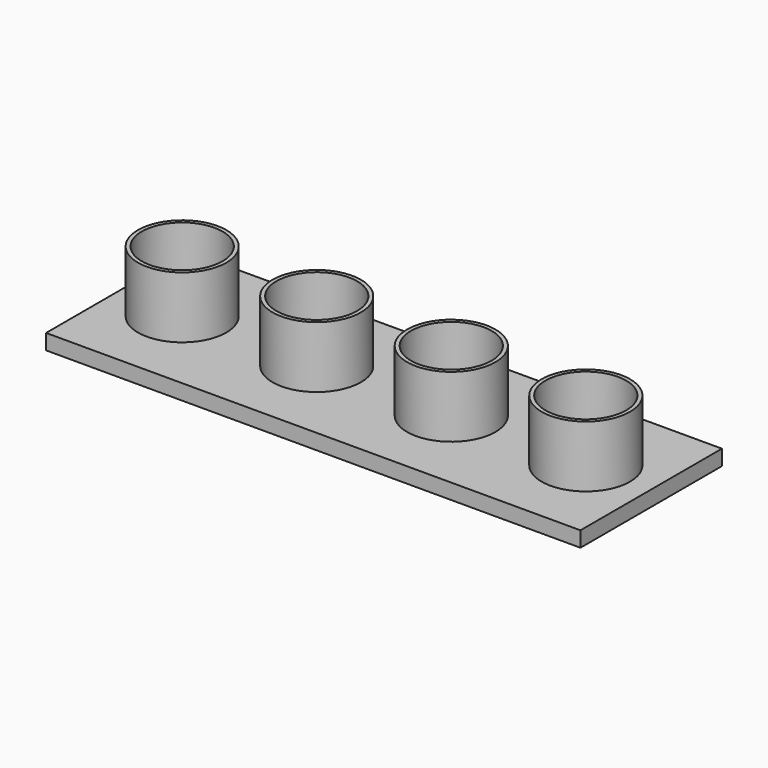
from build123d import *

# Parameters (mm, degrees)
F0_W     = 69.5
F0_H     = 23
F0_R     = 5.75
F0_W_2   = 1
F0_H_2   = 4
F1_DEPTH = 2
F0_R_2   = 5.25
F2_DEPTH = 10


with BuildPart() as f1:
    # F0 (on Top) → F1 (new body)
    with BuildSketch(Plane.XY):
        with Locations((3.4471642077, -3.0003356891)):
            Rectangle(F0_W, F0_H)
        Polygon((-29.8028357923, -13.0003356891), (-29.8028357923, 6.9996643109), (-15.8028357923, 6.9996643109), (-14.8028357923, 6.9996643109), (-13.3028357923, 6.9996643109), (-12.3028357923, 6.9996643109), (1.6971642077, 6.9996643109), (2.6971642077, 6.9996643109), (4.1971642077, 6.9996643109), (5.1971642077, 6.9996643109), (19.1971642077, 6.9996643109), (20.1971642077, 6.9996643109), (21.6971642077, 6.9996643109), (22.6971642077, 6.9996643109), (36.6971642077, 6.9996643109), (36.6971642077, -13.0003356891), (22.6971642077, -13.0003356891), (21.6971642077, -13.0003356891), (20.1971642077, -13.0003356891), (19.1971642077, -13.0003356891), (5.1971642077, -13.0003356891), (5.1971642077, -9.0003356891), (4.1971642077, -9.0003356891), (4.1971642077, -13.0003356891), (2.6971642077, -13.0003356891), (1.6971642077, -13.0003356891), (-12.3028357923, -13.0003356891), (-13.3028357923, -13.0003356891), (-14.8028357923, -13.0003356891), (-15.8028357923, -13.0003356891), align=None, mode=Mode.SUBTRACT)
        Polygon((-15.8028357923, 6.9996643109), (-29.8028357923, 6.9996643109), (-29.8028357923, -13.0003356891), (-15.8028357923, -13.0003356891), (-15.8028357923, -9.0003356891), (-14.8028357923, -9.0003356891), (-14.8028357923, -13.0003356891), (-13.3028357923, -13.0003356891), (-13.3028357923, -9.0003356891), (-12.3028357923, -9.0003356891), (-12.3028357923, -13.0003356891), (1.6971642077, -13.0003356891), (1.6971642077, -9.0003356891), (2.6971642077, -9.0003356891), (2.6971642077, -13.0003356891), (4.1971642077, -13.0003356891), (4.1971642077, -9.0003356891), (5.1971642077, -9.0003356891), (5.1971642077, -13.0003356891), (19.1971642077, -13.0003356891), (19.1971642077, -9.0003356891), (20.1971642077, -9.0003356891), (20.1971642077, -13.0003356891), (21.6971642077, -13.0003356891), (21.6971642077, -9.0003356891), (22.6971642077, -9.0003356891), (22.6971642077, -13.0003356891), (36.6971642077, -13.0003356891), (36.6971642077, 6.9996643109), (22.6971642077, 6.9996643109), (22.6971642077, 2.9996643109), (21.6971642077, 2.9996643109), (21.6971642077, 6.9996643109), (20.1971642077, 6.9996643109), (20.1971642077, 2.9996643109), (19.1971642077, 2.9996643109), (19.1971642077, 6.9996643109), (5.1971642077, 6.9996643109), (5.1971642077, 2.9996643109), (4.1971642077, 2.9996643109), (4.1971642077, 6.9996643109), (2.6971642077, 6.9996643109), (2.6971642077, 2.9996643109), (1.6971642077, 2.9996643109), (1.6971642077, 6.9996643109), (-12.3028357923, 6.9996643109), (-12.3028357923, 2.9996643109), (-13.3028357923, 2.9996643109), (-13.3028357923, 6.9996643109), (-14.8028357923, 6.9996643109), (-14.8028357923, 2.9996643109), (-15.8028357923, 2.9996643109), align=None)
        with Locations((-22.8028357923, -3.0003356891)):
            Circle(F0_R, mode=Mode.SUBTRACT)
        with Locations((-5.3028357923, -3.0003356891)):
            Circle(F0_R, mode=Mode.SUBTRACT)
        with Locations((12.1971642077, -3.0003356891)):
            Circle(F0_R, mode=Mode.SUBTRACT)
        with Locations((29.6971642077, -3.0003356891)):
            Circle(F0_R, mode=Mode.SUBTRACT)
        with Locations((-15.3028357923, 4.9996643109)):
            Rectangle(F0_W_2, F0_H_2)
        with Locations((-12.8028357923, 4.9996643109)):
            Rectangle(F0_W_2, F0_H_2)
        with Locations((2.1971642077, 4.9996643109)):
            Rectangle(F0_W_2, F0_H_2)
        with Locations((4.6971642077, 4.9996643109)):
            Rectangle(F0_W_2, F0_H_2)
        with Locations((19.6971642077, 4.9996643109)):
            Rectangle(F0_W_2, F0_H_2)
        with Locations((22.1971642077, 4.9996643109)):
            Rectangle(F0_W_2, F0_H_2)
        with Locations((-15.3028357923, -11.0003356891)):
            Rectangle(F0_W_2, F0_H_2)
        with Locations((-12.8028357923, -11.0003356891)):
            Rectangle(F0_W_2, F0_H_2)
        with Locations((2.1971642077, -11.0003356891)):
            Rectangle(F0_W_2, F0_H_2)
        with Locations((19.6971642077, -11.0003356891)):
            Rectangle(F0_W_2, F0_H_2)
        with Locations((22.1971642077, -11.0003356891)):
            Rectangle(F0_W_2, F0_H_2)
    extrude(amount=F1_DEPTH)

    # F0 (on Top) → F2 (join)
    with BuildSketch(Plane.XY):
        with Locations((-22.8028357923, -3.0003356891)):
            Circle(F0_R)
        with Locations((-22.8028357923, -3.0003356891)):
            Circle(F0_R_2, mode=Mode.SUBTRACT)
        with Locations((-5.3028357923, -3.0003356891)):
            Circle(F0_R)
        with Locations((-5.3028357923, -3.0003356891)):
            Circle(F0_R_2, mode=Mode.SUBTRACT)
        with Locations((12.1971642077, -3.0003356891)):
            Circle(F0_R)
        with Locations((12.1971642077, -3.0003356891)):
            Circle(F0_R_2, mode=Mode.SUBTRACT)
        with Locations((29.6971642077, -3.0003356891)):
            Circle(F0_R)
        with Locations((29.6971642077, -3.0003356891)):
            Circle(F0_R_2, mode=Mode.SUBTRACT)
    extrude(amount=F2_DEPTH)


solid = f1.part
